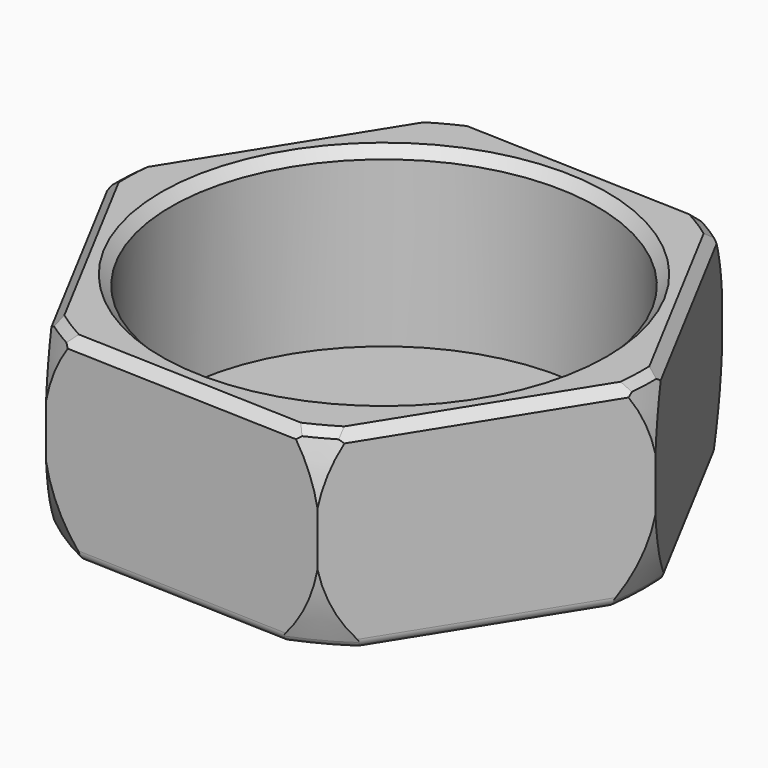
from build123d import *

# Parameters (mm, degrees)
F1_DEPTH     = 2
F2_R         = 22
F3_DEPTH     = 18
F6_T1_DEPTH  = 25.1379794254
F6_T3_DEPTH  = 25.1379794254
F6_T5_DEPTH  = 25.1379794254
F6_T7_DEPTH  = 25.1379794254
F6_T9_DEPTH  = 25.1379794254
F6_T11_DEPTH = 25.1379794254
F6_T14_ANGLE = 28.7689265004
F6_T16_ANGLE = 28.7689265004
F6_T18_ANGLE = 28.7689265004
F6_T20_ANGLE = 28.7689265004
F6_T22_ANGLE = 28.7689265004
F6_T24_ANGLE = 28.7689265004
F7_T1_DEPTH  = 27.9134312771
F7_T3_DEPTH  = 27.9134312771
F7_T5_DEPTH  = 27.9134312771
F7_T7_DEPTH  = 27.9134312771
F7_T9_DEPTH  = 27.9134312771
F7_T11_DEPTH = 27.9134312771
F7_T14_ANGLE = 19.0890287902
F7_T16_ANGLE = 19.0890287902
F7_T18_ANGLE = 19.0890287902
F7_T20_ANGLE = 19.0890287902
F7_T22_ANGLE = 19.0890287902
F7_T24_ANGLE = 19.0890287902


# Not quite as in the source:
# - a fillet or chamfer that OpenCascade refuses, or shapes differently, is made with other operations: its cross-section is extruded or revolved along the edge and cut away or added


with BuildPart() as f1:
    # F0 (on Top) → F1 (new body)
    with BuildSketch(Plane.XY):
        Polygon((13.5351769077, -25.4976924331), (28.8492378388, -1.0270391697), (15.3140609311, 24.4706532633), (-13.5351769077, 25.4976924331), (-28.8492378388, 1.0270391697), (-15.3140609311, -24.4706532633), align=None)
    extrude(amount=F1_DEPTH)

    # F2 (on face) → F3 (join)
    with BuildSketch(Plane.XY.offset(2)):
        Polygon((-15.3140609311, -24.4706532633), (13.5351769077, -25.4976924331), (28.8492378388, -1.0270391697), (15.3140609311, 24.4706532633), (-13.5351769077, 25.4976924331), (-28.8492378388, 1.0270391697), align=None)
        Circle(F2_R, mode=Mode.SUBTRACT)
    extrude(amount=F3_DEPTH)

    # F4 (on Front) → F5 (revolve, cut)
    with BuildSketch(Plane.XZ):
        with BuildLine():
            ThreePointArc((-21.7728036807, -8.449948672), (-27.234187285, 20.6707508781), (-4.2683301811, 39.3900259881))
            Line((-4.2683301811, 39.3900259881), (-38.7757569551, 38.3462198079))
            Line((-38.7757569551, 38.3462198079), (-37.3459825773, -8.9210177113))
            Line((-37.3459825773, -8.9210177113), (-21.7728036807, -8.449948672))
        make_face()
    revolve(axis=Axis((0, 0, 1.6776817089), (0, 0, -1)), mode=Mode.SUBTRACT)

    # F6: fillet of radius 1 on 12 edges, made by hand

    # F6_s2 → F6_t1 (cut)
    with BuildSketch(Plane(origin=(-5.8932508874, 11.1017609583, 0), x_dir=(0, 0, 1), z_dir=(0.4688722819, -0.8832659754, 0))):
        with BuildLine():
            ThreePointArc((1, 25), (0.2928932188, 24.7071067812), (0, 24))
            Line((0, 24), (0, 25))
            Line((0, 25), (1, 25))
        make_face()
    extrude(amount=F6_T1_DEPTH, mode=Mode.SUBTRACT)

    # F6_s4 → F6_t3 (cut)
    with BuildSketch(Plane(origin=(-12.5610324603, 0.4471754998, 0), x_dir=(0, 0, 1), z_dir=(0.9993669139, -0.0355776805, 0))):
        with BuildLine():
            ThreePointArc((0, 24), (0.2928932188, 24.7071067812), (1, 25))
            Line((1, 25), (0, 25))
            Line((0, 25), (0, 24))
        make_face()
    extrude(amount=F6_T3_DEPTH, mode=Mode.SUBTRACT)

    # F6_s6 → F6_t5 (cut)
    with BuildSketch(Plane(origin=(-6.6677815729, -10.6545854585, 0), x_dir=(0, 0, 1), z_dir=(0.5304946321, 0.8476882949, 0))):
        with BuildLine():
            ThreePointArc((0, 24), (0.2928932188, 24.7071067812), (1, 25))
            Line((1, 25), (0, 25))
            Line((0, 25), (0, 24))
        make_face()
    extrude(amount=F6_T5_DEPTH, mode=Mode.SUBTRACT)

    # F6_s8 → F6_t7 (cut)
    with BuildSketch(Plane(origin=(5.8932508874, -11.1017609583, 0), x_dir=(0, 0, 1), z_dir=(-0.4688722819, 0.8832659754, 0))):
        with BuildLine():
            ThreePointArc((0, 24), (0.2928932188, 24.7071067812), (1, 25))
            Line((1, 25), (0, 25))
            Line((0, 25), (0, 24))
        make_face()
    extrude(amount=F6_T7_DEPTH, mode=Mode.SUBTRACT)

    # F6_s10 → F6_t9 (cut)
    with BuildSketch(Plane(origin=(12.5610324603, -0.4471754998, 0), x_dir=(0, 0, 1), z_dir=(-0.9993669139, 0.0355776805, 0))):
        with BuildLine():
            ThreePointArc((0, 24), (0.2928932188, 24.7071067812), (1, 25))
            Line((1, 25), (0, 25))
            Line((0, 25), (0, 24))
        make_face()
    extrude(amount=F6_T9_DEPTH, mode=Mode.SUBTRACT)

    # F6_s12 → F6_t11 (cut)
    with BuildSketch(Plane(origin=(6.6677815729, 10.6545854585, 0), x_dir=(0, 0, 1), z_dir=(-0.5304946321, -0.8476882949, 0))):
        with BuildLine():
            ThreePointArc((0, 24), (0.2928932188, 24.7071067812), (1, 25))
            Line((1, 25), (0, 25))
            Line((0, 25), (0, 24))
        make_face()
    extrude(amount=F6_T11_DEPTH, mode=Mode.SUBTRACT)

    # F6_s13 → F6_t14 (revolve, cut)
    with BuildSketch(Plane(origin=(0, 0, 0), x_dir=(0, 0, 1), z_dir=(0.2827322942, 0.9591988583, 0))):
        with BuildLine():
            ThreePointArc((0.6533621298, -27.201971973), (0.179439865, -26.8355331418), (0, -26.2639729395))
            Line((0, -26.2639729395), (0, -26.9515222916))
            ThreePointArc((0, -26.9515222916), (0.3259256733, -27.0787177648), (0.6533621298, -27.201971973))
        make_face()
    revolve(axis=Axis((0, 0, 0), (0, 0, 1)), revolution_arc=F6_T14_ANGLE, mode=Mode.SUBTRACT)

    # F6_s15 → F6_t16 (revolve, cut)
    with BuildSketch(Plane(origin=(0, 0, 0), x_dir=(0, 0, 1), z_dir=(-0.6893244315, 0.7244527784, 0))):
        with BuildLine():
            ThreePointArc((0, -26.2639729395), (0.179439865, -26.8355331418), (0.6533621298, -27.201971973))
            ThreePointArc((0.6533621298, -27.201971973), (0.3259256733, -27.0787177648), (0, -26.9515222916))
            Line((0, -26.9515222916), (0, -26.2639729395))
        make_face()
    revolve(axis=Axis((0, 0, 0), (0, 0, 1)), revolution_arc=F6_T16_ANGLE, mode=Mode.SUBTRACT)

    # F6_s17 → F6_t18 (revolve, cut)
    with BuildSketch(Plane(origin=(0, 0, 0), x_dir=(0, 0, 1), z_dir=(-0.9720567257, -0.2347460799, 0))):
        with BuildLine():
            ThreePointArc((0, -26.2639729395), (0.179439865, -26.8355331418), (0.6533621298, -27.201971973))
            ThreePointArc((0.6533621298, -27.201971973), (0.3259256733, -27.0787177648), (0, -26.9515222916))
            Line((0, -26.9515222916), (0, -26.2639729395))
        make_face()
    revolve(axis=Axis((0, 0, 0), (0, 0, 1)), revolution_arc=F6_T18_ANGLE, mode=Mode.SUBTRACT)

    # F6_s19 → F6_t20 (revolve, cut)
    with BuildSketch(Plane(origin=(0, 0, 0), x_dir=(0, 0, 1), z_dir=(-0.2827322942, -0.9591988583, 0))):
        with BuildLine():
            ThreePointArc((0, -26.2639729395), (0.179439865, -26.8355331418), (0.6533621298, -27.201971973))
            ThreePointArc((0.6533621298, -27.201971973), (0.3259256733, -27.0787177648), (0, -26.9515222916))
            Line((0, -26.9515222916), (0, -26.2639729395))
        make_face()
    revolve(axis=Axis((0, 0, 0), (0, 0, 1)), revolution_arc=F6_T20_ANGLE, mode=Mode.SUBTRACT)

    # F6_s21 → F6_t22 (revolve, cut)
    with BuildSketch(Plane(origin=(0, 0, 0), x_dir=(0, 0, 1), z_dir=(0.6893244315, -0.7244527784, 0))):
        with BuildLine():
            ThreePointArc((0, -26.2639729395), (0.179439865, -26.8355331418), (0.6533621298, -27.201971973))
            ThreePointArc((0.6533621298, -27.201971973), (0.3259256733, -27.0787177648), (0, -26.9515222916))
            Line((0, -26.9515222916), (0, -26.2639729395))
        make_face()
    revolve(axis=Axis((0, 0, 0), (0, 0, 1)), revolution_arc=F6_T22_ANGLE, mode=Mode.SUBTRACT)

    # F6_s23 → F6_t24 (revolve, cut)
    with BuildSketch(Plane(origin=(0, 0, 0), x_dir=(0, 0, 1), z_dir=(0.9720567257, 0.2347460799, 0))):
        with BuildLine():
            ThreePointArc((0, -26.2639729395), (0.179439865, -26.8355331418), (0.6533621298, -27.201971973))
            ThreePointArc((0.6533621298, -27.201971973), (0.3259256733, -27.0787177648), (0, -26.9515222916))
            Line((0, -26.9515222916), (0, -26.2639729395))
        make_face()
    revolve(axis=Axis((0, 0, 0), (0, 0, 1)), revolution_arc=F6_T24_ANGLE, mode=Mode.SUBTRACT)

    # F7: chamfer of 1 on 13 edges, made by hand

    # F7_s2 → F7_t1 (cut)
    with BuildSketch(Plane(origin=(-6.5439171089, 12.3274920518, 0), x_dir=(0, 0, 1), z_dir=(0.4688722819, -0.8832659754, 0))):
        Polygon((19, 25), (20, 24), (20, 25), align=None)
    extrude(amount=F7_T1_DEPTH, mode=Mode.SUBTRACT)

    # F7_s4 → F7_t3 (cut)
    with BuildSketch(Plane(origin=(-13.9478798363, 0.4965475694, 0), x_dir=(0, 0, 1), z_dir=(0.9993669139, -0.0355776805, 0))):
        Polygon((19, 25), (20, 24), (20, 25), align=None)
    extrude(amount=F7_T3_DEPTH, mode=Mode.SUBTRACT)

    # F7_s6 → F7_t5 (cut)
    with BuildSketch(Plane(origin=(-7.4039627274, -11.8309444824, 0), x_dir=(0, 0, 1), z_dir=(0.5304946321, 0.8476882949, 0))):
        Polygon((20, 24), (19, 25), (20, 25), align=None)
    extrude(amount=F7_T5_DEPTH, mode=Mode.SUBTRACT)

    # F7_s8 → F7_t7 (cut)
    with BuildSketch(Plane(origin=(6.5439171089, -12.3274920518, 0), x_dir=(0, 0, 1), z_dir=(-0.4688722819, 0.8832659754, 0))):
        Polygon((20, 24), (19, 25), (20, 25), align=None)
    extrude(amount=F7_T7_DEPTH, mode=Mode.SUBTRACT)

    # F7_s10 → F7_t9 (cut)
    with BuildSketch(Plane(origin=(13.9478798363, -0.4965475694, 0), x_dir=(0, 0, 1), z_dir=(-0.9993669139, 0.0355776805, 0))):
        Polygon((20, 24), (19, 25), (20, 25), align=None)
    extrude(amount=F7_T9_DEPTH, mode=Mode.SUBTRACT)

    # F7_s12 → F7_t11 (cut)
    with BuildSketch(Plane(origin=(7.4039627274, 11.8309444824, 0), x_dir=(0, 0, 1), z_dir=(-0.5304946321, -0.8476882949, 0))):
        Polygon((19, 25), (20, 24), (20, 25), align=None)
    extrude(amount=F7_T11_DEPTH, mode=Mode.SUBTRACT)

    # F7_s13 → F7_t14 (revolve, cut)
    with BuildSketch(Plane(origin=(0, 0, 0), x_dir=(0, 0, 1), z_dir=(0.2007940306, 0.9796334811, 0))):
        with BuildLine():
            Line((20, -26.7433589462), (19.2962192727, -27.6984789085))
            ThreePointArc((19.2962192727, -27.6984789085), (19.6333817199, -27.5916538552), (20, -27.4703288742))
            Line((20, -27.4703288742), (20, -26.7433589462))
        make_face()
    revolve(axis=Axis((0, 0, 20), (0, 0, 1)), revolution_arc=F7_T14_ANGLE, mode=Mode.SUBTRACT)

    # F7_s15 → F7_t16 (revolve, cut)
    with BuildSketch(Plane(origin=(0, 0, 0), x_dir=(0, 0, 1), z_dir=(-0.7479904657, 0.663709472, 0))):
        with BuildLine():
            Line((19.2962192727, -27.6984789085), (20, -26.7433589462))
            Line((20, -26.7433589462), (20, -27.4703288742))
            ThreePointArc((20, -27.4703288742), (19.6333817199, -27.5916538552), (19.2962192727, -27.6984789085))
        make_face()
    revolve(axis=Axis((0, 0, 20), (0, 0, 1)), revolution_arc=F7_T16_ANGLE, mode=Mode.SUBTRACT)

    # F7_s17 → F7_t18 (revolve, cut)
    with BuildSketch(Plane(origin=(0, 0, 0), x_dir=(0, 0, 1), z_dir=(-0.9487844963, -0.3159240091, 0))):
        with BuildLine():
            Line((20, -26.7433589462), (19.2962192727, -27.6984789085))
            ThreePointArc((19.2962192727, -27.6984789085), (19.6333817199, -27.5916538552), (20, -27.4703288742))
            Line((20, -27.4703288742), (20, -26.7433589462))
        make_face()
    revolve(axis=Axis((0, 0, 20), (0, 0, 1)), revolution_arc=F7_T18_ANGLE, mode=Mode.SUBTRACT)

    # F7_s19 → F7_t20 (revolve, cut)
    with BuildSketch(Plane(origin=(0, 0, 0), x_dir=(0, 0, 1), z_dir=(-0.2007940306, -0.9796334811, 0))):
        with BuildLine():
            Line((20, -26.7433589462), (19.2962192727, -27.6984789085))
            ThreePointArc((19.2962192727, -27.6984789085), (19.6333817199, -27.5916538552), (20, -27.4703288742))
            Line((20, -27.4703288742), (20, -26.7433589462))
        make_face()
    revolve(axis=Axis((0, 0, 20), (0, 0, 1)), revolution_arc=F7_T20_ANGLE, mode=Mode.SUBTRACT)

    # F7_s21 → F7_t22 (revolve, cut)
    with BuildSketch(Plane(origin=(0, 0, 0), x_dir=(0, 0, 1), z_dir=(0.7479904657, -0.663709472, 0))):
        with BuildLine():
            Line((20, -26.7433589462), (19.2962192727, -27.6984789085))
            ThreePointArc((19.2962192727, -27.6984789085), (19.6333817199, -27.5916538552), (20, -27.4703288742))
            Line((20, -27.4703288742), (20, -26.7433589462))
        make_face()
    revolve(axis=Axis((0, 0, 20), (0, 0, 1)), revolution_arc=F7_T22_ANGLE, mode=Mode.SUBTRACT)

    # F7_s23 → F7_t24 (revolve, cut)
    with BuildSketch(Plane(origin=(0, 0, 0), x_dir=(0, 0, 1), z_dir=(0.9487844963, 0.3159240091, 0))):
        with BuildLine():
            Line((20, -26.7433589462), (19.2962192727, -27.6984789085))
            ThreePointArc((19.2962192727, -27.6984789085), (19.6333817199, -27.5916538552), (20, -27.4703288742))
            Line((20, -27.4703288742), (20, -26.7433589462))
        make_face()
    revolve(axis=Axis((0, 0, 20), (0, 0, 1)), revolution_arc=F7_T24_ANGLE, mode=Mode.SUBTRACT)

    # F7_s25 → F7_t26 (revolve, cut)
    with BuildSketch(Plane.XZ):
        Polygon((23, 20), (22, 19), (22, 20), align=None)
    revolve(axis=Axis((0, 0, 20), (0, 0, 1)), mode=Mode.SUBTRACT)


solid = f1.part
